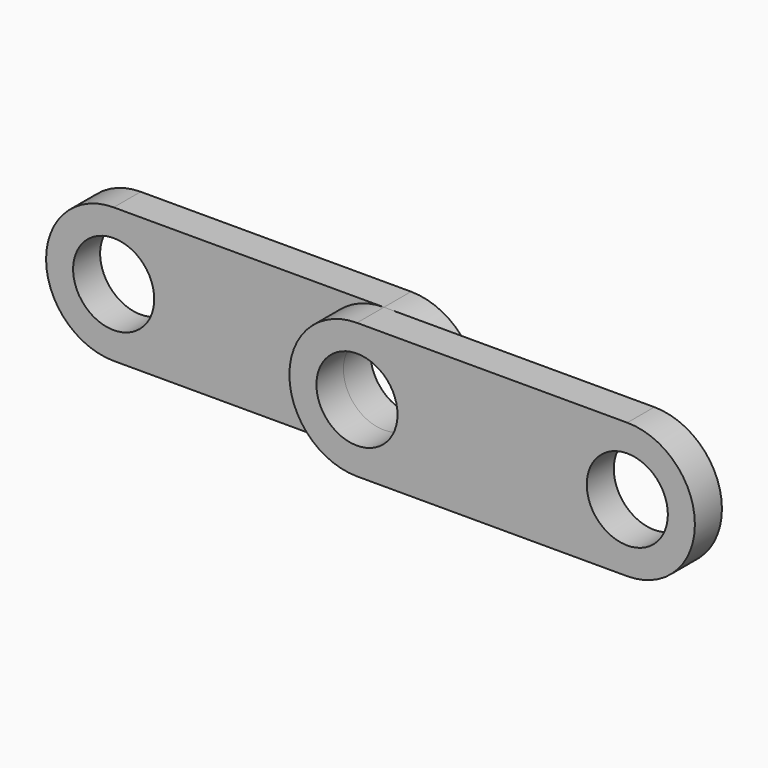
from build123d import *

# Parameters (mm, degrees)
F0_R     = 6
F1_DEPTH = 5
F2_R     = 6
F3_DEPTH = 5


# Not quite as in the source:
# - the program builds the solid bodies; features that only make, move or delete a surface that nothing else refers to are left out


with BuildPart() as f1:
    # F0 (on Front) → F1 (new body)
    with BuildSketch(Plane.XZ):
        with BuildLine():
            ThreePointArc((-8.4734316129, -10), (1.5265683871, 2.052e-07), (-8.4734320234, 10))
            Line((-8.4734320234, 10), (-48.4734320234, 10))
            ThreePointArc((-48.4734320234, 10), (-58.4734320234, 0), (-48.4734320234, -10))
            Line((-48.4734320234, -10), (-8.4734316129, -10))
        make_face()
        with Locations((-48.4734320234, 0)):
            Circle(F0_R, mode=Mode.SUBTRACT)
        with Locations((-8.4734320234, 0)):
            Circle(F0_R, mode=Mode.SUBTRACT)
    extrude(amount=F1_DEPTH)

    # F2 (on face) → F3 (join)
    with BuildSketch(Plane.XZ.offset(5)):
        with BuildLine():
            ThreePointArc((31.5265687976, -10), (41.5265687976, 2.052e-07), (31.5265683871, 10))
            Line((31.5265683871, 10), (-8.4734316129, 10))
            ThreePointArc((-8.4734316129, 10), (-18.4734316129, 0), (-8.4734316129, -10))
            Line((-8.4734316129, -10), (31.5265687976, -10))
        make_face()
        with Locations((-8.4734316129, 0)):
            Circle(F2_R, mode=Mode.SUBTRACT)
        with Locations((31.5265683871, 0)):
            Circle(F2_R, mode=Mode.SUBTRACT)
    extrude(amount=F3_DEPTH)


solid = f1.part
